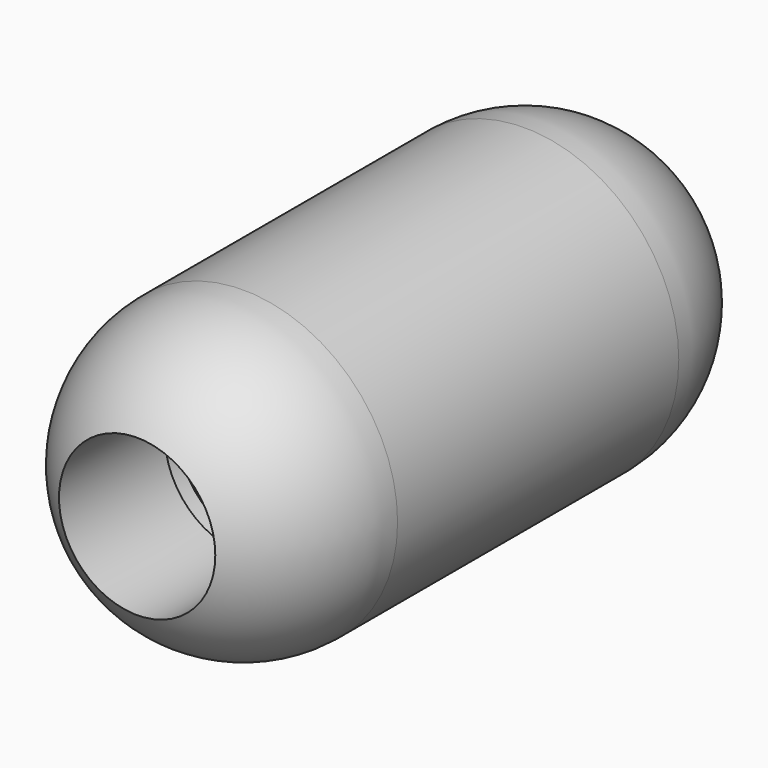
from build123d import *

# Parameters (mm, degrees)
F0_R     = 4.7625
F1_DEPTH = 19.05
F4_R     = 2.413
F5_DEPTH = 19.051
F8_R     = 2.54
F9_DEPTH = 0.6096


# Not quite as in the source:
# - a fillet or chamfer that OpenCascade refuses, or shapes differently, is made with other operations: its cross-section is extruded or revolved along the edge and cut away or added


with BuildPart() as f1:
    # F0 (on Front) → F1 (new body)
    with BuildSketch(Plane.XZ):
        Circle(F0_R)
    extrude(amount=F1_DEPTH)

    # F4 (on face) → F5 (cut, through all)
    with BuildSketch(Plane.XZ):
        Circle(F4_R)
    extrude(amount=F5_DEPTH, mode=Mode.SUBTRACT)

    # F6: fillet of radius 4.7498 on 2 edges, made by hand

    # F6_s1 → F6_t2 (revolve, cut)
    with BuildSketch(Plane.XY):
        with BuildLine():
            ThreePointArc((4.7625, -4.0986778295), (4.1334732879, -1.7365119695), (2.413, 0))
            Line((2.413, 0), (4.7625, 0))
            Line((4.7625, 0), (4.7625, -4.0986778295))
        make_face()
    revolve(axis=Axis((0, 0, 0), (0, -1, 0)), mode=Mode.SUBTRACT)

    # F6_s3 → F6_t4 (revolve, cut)
    with BuildSketch(Plane.XY):
        with BuildLine():
            ThreePointArc((4.7625, -14.9513221705), (4.1334732879, -17.3134880305), (2.413, -19.05))
            Line((2.413, -19.05), (4.7625, -19.05))
            Line((4.7625, -19.05), (4.7625, -14.9513221705))
        make_face()
    revolve(axis=Axis((0, -19.05, 0), (0, -1, 0)), mode=Mode.SUBTRACT)

    # F8 (on offset) → F9 (cut)
    with BuildSketch(Plane.XZ.offset(14.9606)):
        Circle(F8_R)
    extrude(amount=-F9_DEPTH, mode=Mode.SUBTRACT)


solid = f1.part
